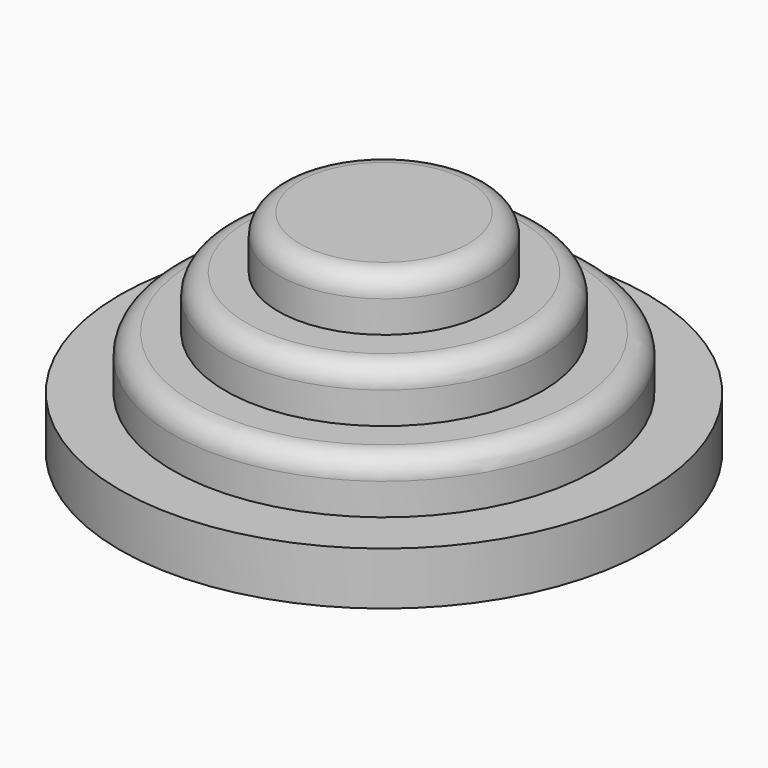
from build123d import *

# Parameters (mm, degrees)
F0_R     = 63.5
F1_DEPTH = 12.7
F4_R     = 50.8
F5_DEPTH = 25.4
F6_R     = 38.1
F7_DEPTH = 38.1
F8_R     = 25.4
F9_DEPTH = 50.8
F10_R    = 5.08
F11_R    = 5.08
F12_R    = 5.08


# Not quite as in the source:
# - the program builds the solid bodies; features that only make, move or delete a surface that nothing else refers to are left out


with BuildPart() as f1:
    # F0 (on Top) → F1 (new body)
    with BuildSketch(Plane.XY):
        Circle(F0_R)
    extrude(amount=F1_DEPTH)

    # F4 (on Top) → F5 (join)
    with BuildSketch(Plane.XY):
        Circle(F4_R)
    extrude(amount=F5_DEPTH)

    # F6 (on Top) → F7 (join)
    with BuildSketch(Plane.XY):
        Circle(F6_R)
    extrude(amount=F7_DEPTH)

    # F8 (on Top) → F9 (join)
    with BuildSketch(Plane.XY):
        Circle(F8_R)
    extrude(amount=F9_DEPTH)

    # F10
    f10_edges = [f1.edges().sort_by_distance(p)[0] for p in [
        (-25.4, 0, 50.8),
    ]]
    fillet(f10_edges, radius=F10_R)

    # F11
    f11_edges = [f1.edges().sort_by_distance(p)[0] for p in [
        (-38.1, 0, 38.1),
    ]]
    fillet(f11_edges, radius=F11_R)

    # F12
    f12_edges = [f1.edges().sort_by_distance(p)[0] for p in [
        (-50.8, 0, 25.4),
    ]]
    fillet(f12_edges, radius=F12_R)


solid = f1.part
